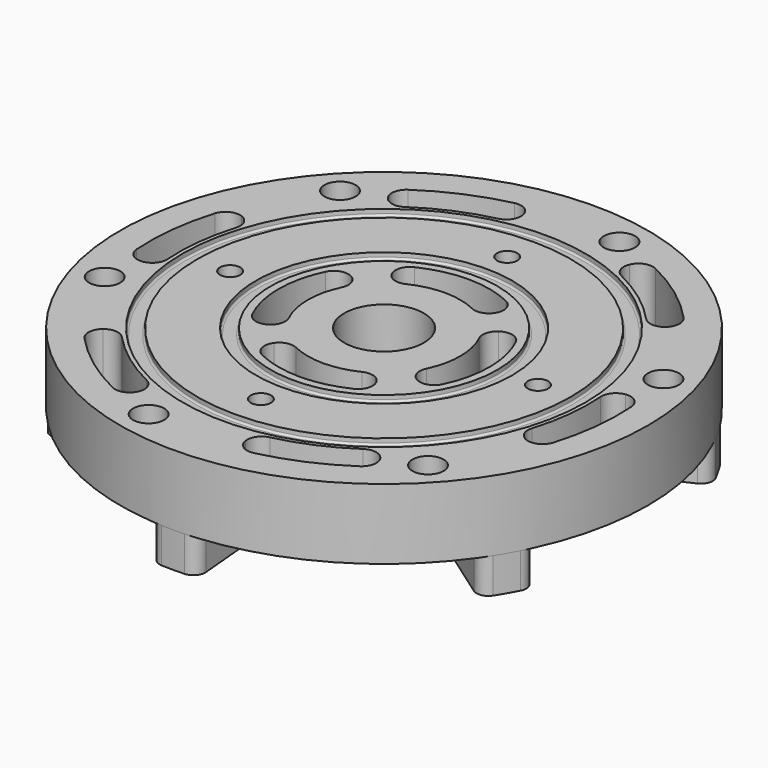
from build123d import *

# Parameters (mm, degrees)
F0_R             = 57.15
F1_DEPTH         = 15.24
F2_R             = 8.636
F3_DEPTH         = 15.241
F5_DEPTH         = 7.62
F6_T1_DEPTH      = 14.2671475518
F6_T3_DEPTH      = 13.7344913133
F8_COUNT         = 6
F9_D             = 4.3942
F9_DEPTH         = 15.24
F9_TIP           = 1.3201508661
F10_R            = 43.6245
F10_R_2          = 40.4241
F11_DEPTH        = 1.2954
F12_R            = 0.4064
F14_DEPTH        = 22.861
F14_COPIES_COUNT = 6
F15_R            = 3.17499
F16_R            = 27.7495
F16_R_2          = 24.5491
F17_DEPTH        = 1.2954
F18_R            = 0.4064
F20_DEPTH        = 22.861
F20_COPIES_COUNT = 4
F21_R            = 3.17499
F23_D            = 4.3942
F23_DEPTH        = 6.35
F23_TIP          = 1.3201508661
F25_D            = 6.7564


# Not quite as in the source:
# - a fillet or chamfer that OpenCascade refuses, or shapes differently, is made with other operations: its cross-section is extruded or revolved along the edge and cut away or added
# - a fillet or chamfer is up to 0.001 mm smaller than in the source, because OpenCascade refuses the exact size
# - a pattern or mirror of a feature is missing from the dataset's text; its kind, count and spacing are read off the source's solid


with BuildPart() as f1:
    # F0 (on Top) → F1 (new body)
    with BuildSketch(Plane.XY):
        Circle(F0_R)
    extrude(amount=F1_DEPTH)

    # F2 (on face) → F3 (cut, through all)
    with BuildSketch(Plane.XY.offset(15.24)):
        Circle(F2_R)
    extrude(amount=-F3_DEPTH, mode=Mode.SUBTRACT)

    # F4 (on face) → F5 (join)
    with BuildSketch(Plane(origin=(0, 0, 0), x_dir=(1, 0, 0), z_dir=(0, 0, -1))):
        with BuildLine():
            Line((-2.8575, -31.6211510504), (-5.1435, -56.9180718907))
            ThreePointArc((-5.1435, -56.9180718907), (0, -57.15), (5.1435, -56.9180718907))
            Line((5.1435, -56.9180718907), (2.8575, -31.6211510504))
            ThreePointArc((2.8575, -31.6211510504), (0, -31.75), (-2.8575, -31.6211510504))
        make_face()
    extrude(amount=F5_DEPTH)

    # F6: fillet of radius 2.54 on 4 edges, made by hand

    # F6_s2 → F6_t1 (cut)
    with BuildSketch(Plane.XY.offset(-14.2671475518)):
        with BuildLine():
            ThreePointArc((2.490581259, 57.0957047858), (4.2919178251, 56.2301660065), (4.9095808426, 54.3295179065))
            Line((4.9095808426, 54.3295179065), (5.1435, 56.9180718907))
            ThreePointArc((5.1435, 56.9180718907), (3.8180737982, 57.022318547), (2.490581259, 57.0957047858))
        make_face()
        with BuildLine():
            ThreePointArc((-2.490581259, 57.0957047858), (-4.2919178251, 56.2301660065), (-4.9095808426, 54.3295179065))
            Line((-4.9095808426, 54.3295179065), (-5.1435, 56.9180718907))
            ThreePointArc((-5.1435, 56.9180718907), (-3.8180737982, 57.022318547), (-2.490581259, 57.0957047858))
        make_face()
    extrude(amount=F6_T1_DEPTH, mode=Mode.SUBTRACT)

    # F6_s4 → F6_t3 (cut)
    with BuildSketch(Plane.XY.offset(-13.7344913133)):
        with BuildLine():
            ThreePointArc((0.5073422252, 31.7459462588), (2.2462164703, 32.396860006), (3.0776216873, 34.0570219595))
            Line((3.0776216873, 34.0570219595), (2.8575, 31.6211510504))
            ThreePointArc((2.8575, 31.6211510504), (1.6835778156, 31.7053318188), (0.5073422252, 31.7459462588))
        make_face()
        with BuildLine():
            ThreePointArc((-3.0776216873, 34.0570219595), (-2.2462164703, 32.396860006), (-0.5073422252, 31.7459462588))
            ThreePointArc((-0.5073422252, 31.7459462588), (-1.6835778156, 31.7053318188), (-2.8575, 31.6211510504))
            Line((-2.8575, 31.6211510504), (-3.0776216873, 34.0570219595))
        make_face()
    extrude(amount=F6_T3_DEPTH, mode=Mode.SUBTRACT)

    # F8: F1 ×6 about axis
    f8_axis = Axis((0, 0, 15.24), (0, 0, 1))


with BuildPart() as f1_1:
    add(f1.part)
    for i in range(1, F8_COUNT):
        add(f1.part.rotate(f8_axis, i * 360 / F8_COUNT))

    # F9
    with Locations(Plane(origin=(0, 0, -7.62), x_dir=(1, 0, 0), z_dir=(0, 0, -1))):
        with Locations((0, -50.8), (43.9940905122, -25.4), (43.9940905122, 25.4), (0, 50.8), (-43.9940905122, 25.4), (-43.9940905122, -25.4)):
            Hole(F9_D / 2, depth=F9_DEPTH)
            with Locations((0, 0, -(F9_DEPTH + F9_TIP / 2))):  # 118° drill point
                Cone(0, F9_D / 2, F9_TIP, mode=Mode.SUBTRACT)

    # F10 (on face) → F11 (cut)
    with BuildSketch(Plane.XY.offset(15.24)):
        Circle(F10_R)
        Circle(F10_R_2, mode=Mode.SUBTRACT)
    extrude(amount=-F11_DEPTH, mode=Mode.SUBTRACT)

    # F12
    f12_edges = [f1_1.edges().sort_by_distance(p)[0] for p in [
        (-43.6245, 0, 13.9446),
        (-40.4241, 0, 13.9446),
    ]]
    fillet(f12_edges, radius=F12_R)

    # F13 (on face) → F14 (cut, through all)
    with BuildSketch(Plane.XY.offset(15.24)):
        with BuildLine():
            ThreePointArc((16.721010174, 41.1850739803), (26.4387827868, 35.7322440487), (34.49502146, 28.0338365993))
            Line((34.49502146, 28.0338365993), (39.4228816685, 32.0386703992))
            ThreePointArc((39.4228816685, 32.0386703992), (30.2157517563, 40.8368503413), (19.1097259131, 47.0686559775))
            Line((19.1097259131, 47.0686559775), (16.721010174, 41.1850739803))
        make_face()
    f14 = extrude(amount=-F14_DEPTH, mode=Mode.SUBTRACT)

    # F14_copies: F14 ×6 about axis
    f14_copies_axis = Axis((0, 0, 0), (0, 0, 1))
    for i in range(1, F14_COPIES_COUNT):
        add(f14.rotate(f14_copies_axis, i * 360 / F14_COPIES_COUNT), mode=Mode.SUBTRACT)

    # F15 (radius 3.175 in the source; OpenCascade refuses exactly that, so slightly less here)
    f15_edges = [f1_1.edges().sort_by_distance(p)[0] for p in [
        (39.422882, 32.03867, 7.62),
        (19.109726, 47.068656, 7.62),
        (16.72101, 41.185074, 7.62),
        (34.495021, 28.033837, 7.62),
    ]]
    fillet(f15_edges, radius=F15_R)

    # F16 (on face) → F17 (cut)
    with BuildSketch(Plane.XY.offset(15.24)):
        Circle(F16_R)
        Circle(F16_R_2, mode=Mode.SUBTRACT)
    extrude(amount=-F17_DEPTH, mode=Mode.SUBTRACT)

    # F18
    f18_edges = [f1_1.edges().sort_by_distance(p)[0] for p in [
        (-27.7495, 0, 13.9446),
        (-24.5491, 0, 13.9446),
    ]]
    fillet(f18_edges, radius=F18_R)

    # F19 (on face) → F20 (cut, through all)
    with BuildSketch(Plane.XY.offset(15.24)):
        with BuildLine():
            Line((13.111957335, -18.7258157324), (9.4697469642, -13.5242002512))
            ThreePointArc((9.4697469642, -13.5242002512), (0, -16.51), (-9.4697469642, -13.5242002512))
            Line((-9.4697469642, -13.5242002512), (-13.111957335, -18.7258157324))
            ThreePointArc((-13.111957335, -18.7258157324), (0, -22.86), (13.111957335, -18.7258157324))
        make_face()
    f20 = extrude(amount=-F20_DEPTH, mode=Mode.SUBTRACT)

    # F20_copies: F20 ×4 about axis
    f20_copies_axis = Axis((0, 0, 0), (0, 0, 1))
    for i in range(1, F20_COPIES_COUNT):
        add(f20.rotate(f20_copies_axis, i * 360 / F20_COPIES_COUNT), mode=Mode.SUBTRACT)

    # F21 (radius 3.175 in the source; OpenCascade refuses exactly that, so slightly less here)
    f21_edges = [f1_1.edges().sort_by_distance(p)[0] for p in [
        (-9.469747, -13.5242, 7.62),
        (-13.111957, -18.725816, 7.62),
        (9.469747, -13.5242, 7.62),
        (13.111957, -18.725816, 7.62),
        (-13.5242, -9.469747, 7.62),
        (-18.725816, -13.111957, 7.62),
        (-13.5242, 9.469747, 7.62),
        (-18.725816, 13.111957, 7.62),
        (13.5242, 9.469747, 7.62),
        (18.725816, 13.111957, 7.62),
        (18.725816, -13.111957, 7.62),
        (13.5242, -9.469747, 7.62),
        (-9.469747, 13.5242, 7.62),
        (-13.111957, 18.725816, 7.62),
        (13.111957, 18.725816, 7.62),
        (9.469747, 13.5242, 7.62),
        (-16.72101, -41.185074, 7.62),
        (-19.109726, -47.068656, 7.62),
        (-39.422882, -32.03867, 7.62),
        (-34.495021, -28.033837, 7.62),
        (27.306815, -35.073357, 7.62),
        (31.207789, -40.083836, 7.62),
        (8.034862, -50.160552, 7.62),
        (7.030504, -43.890483, 7.62),
        (44.027825, 6.111717, 7.62),
        (50.317515, 6.98482, 7.62),
        (47.457743, -18.121882, 7.62),
        (41.525525, -15.856647, 7.62),
        (-44.027825, -6.111717, 7.62),
        (-50.317515, -6.98482, 7.62),
        (-47.457743, 18.121882, 7.62),
        (-41.525525, 15.856647, 7.62),
        (-27.306815, 35.073357, 7.62),
        (-31.207789, 40.083836, 7.62),
        (-8.034862, 50.160552, 7.62),
        (-7.030504, 43.890483, 7.62),
    ]]
    fillet(f21_edges, radius=F21_R)

    # F23
    with Locations(Plane.XY.offset(15.24)):
        with Locations((-33.3375, 0), (0, -33.3375), (33.3375, 0), (0, 33.3375)):
            Hole(F23_D / 2, depth=F23_DEPTH)
            with Locations((0, 0, -(F23_DEPTH + F23_TIP / 2))):  # 118° drill point
                Cone(0, F23_D / 2, F23_TIP, mode=Mode.SUBTRACT)

    # F25 (through all)
    with Locations(Plane.XY.offset(15.24)):
        with Locations((11.3576544358, 49.5140756323), (48.5592745603, 14.9210205473), (37.2016201245, -34.593055085), (-11.3576544358, -49.5140756323), (-48.5592745603, -14.9210205473), (-37.2016201245, 34.593055085)):
            Hole(F25_D / 2)


solid = f1_1.part
